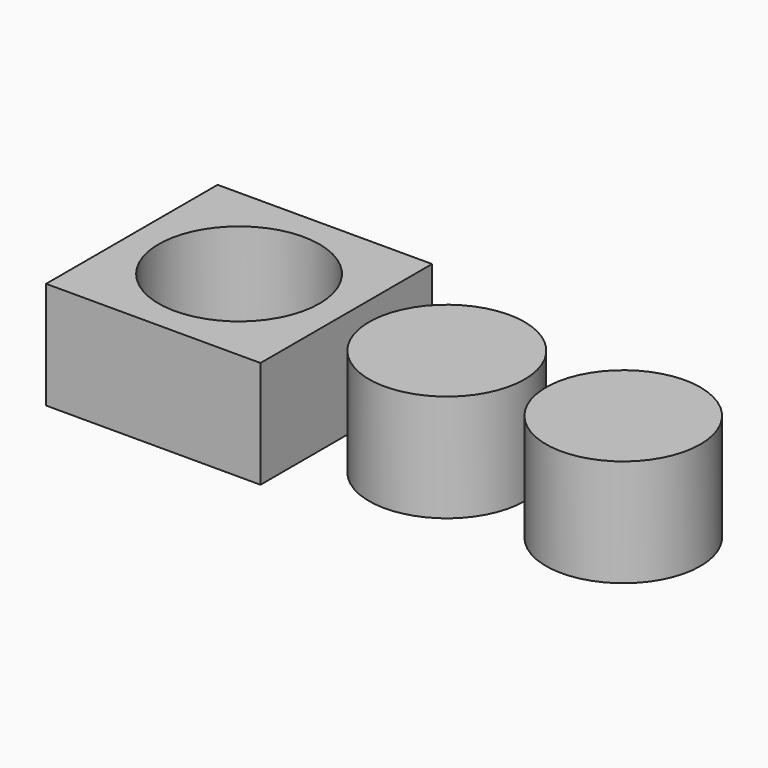
from build123d import *

# Parameters (mm, degrees)
F0_W     = 20
F0_H     = 20
F0_R     = 7.5
F1_DEPTH = 10
F0_R_2   = 7.2
F0_R_3   = 7.25


# Not quite as in the source:
# - a feature names something its author has since deleted; it is built from what else it names


with BuildPart() as f1:
    # F0 (on Top) → F1 (new body)
    with BuildSketch(Plane.XY):
        Rectangle(F0_W, F0_H)
        Circle(F0_R, mode=Mode.SUBTRACT)
    extrude(amount=F1_DEPTH)


with BuildPart() as f1b:
    # F0 (on Top) → F1, piece 2 (new body)
    with BuildSketch(Plane.XY):
        with Locations((35.8341895044, 0)):
            Circle(F0_R_2)
    extrude(amount=F1_DEPTH)


with BuildPart() as f1c:
    # F0 (on Top) → F1, piece 3 (new body)
    with BuildSketch(Plane.XY):
        with Locations((19.3803589791, 0)):
            Circle(F0_R_3)
    extrude(amount=F1_DEPTH)


solid = Compound([f1.part, f1b.part, f1c.part])
